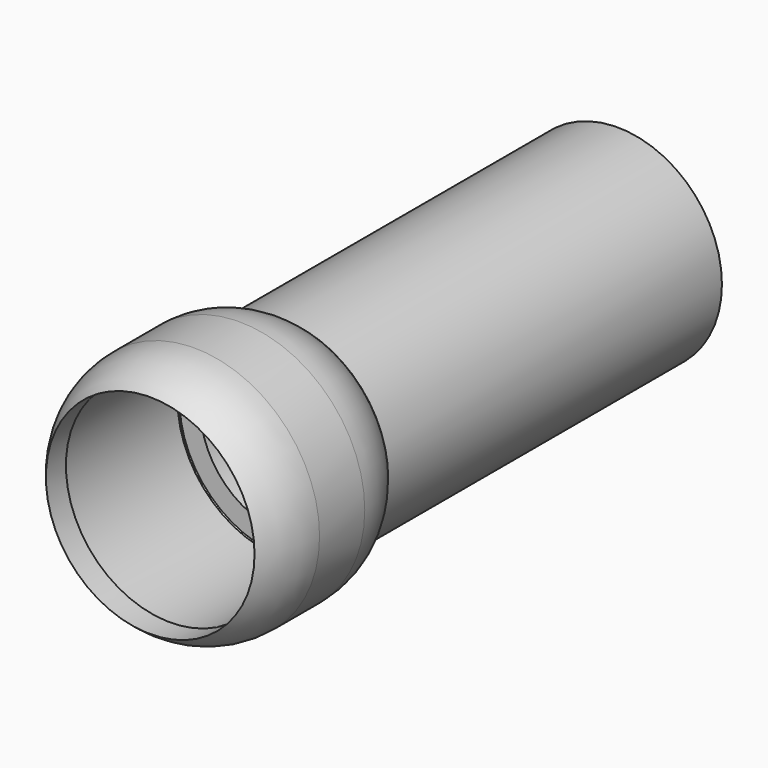
from build123d import *

# Parameters (mm, degrees)
F0_R     = 38.1
F0_R_2   = 31.75
F1_DEPTH = 50.8
F4_R     = 32.0360083413
F5_DEPTH = 43.18
F6_R     = 31.75
F6_R_2   = 25.4
F7_DEPTH = 127


# Not quite as in the source:
# - a fillet or chamfer that OpenCascade refuses, or shapes differently, is made with other operations: its cross-section is extruded or revolved along the edge and cut away or added


with BuildPart() as f1:
    # F0 (on Front) → F1 (new body)
    with BuildSketch(Plane.XZ):
        Circle(F0_R)
        Circle(F0_R_2, mode=Mode.SUBTRACT)
    extrude(amount=F1_DEPTH)

    # F2: fillet of radius 25.4 on 1 edges, made by hand

    # F2_s1 → F2_t2 (revolve, cut)
    with BuildSketch(Plane.XY):
        with BuildLine():
            ThreePointArc((38.1, -33.9994791747), (36.459524406, -42.9797352958), (31.75, -50.8))
            Line((31.75, -50.8), (38.1, -50.8))
            Line((38.1, -50.8), (38.1, -33.9994791747))
        make_face()
    revolve(axis=Axis((0, -50.8, 0), (0, -1, 0)), mode=Mode.SUBTRACT)

    # F3: fillet of radius 25.4 on 1 edges, made by hand

    # F3_s1 → F3_t2 (revolve, cut)
    with BuildSketch(Plane.XY):
        with BuildLine():
            ThreePointArc((38.1, -16.8005208253), (36.459524406, -7.8202647042), (31.75, 0))
            Line((31.75, 0), (38.1, 0))
            Line((38.1, 0), (38.1, -16.8005208253))
        make_face()
    revolve(axis=Axis((0, 0, 0), (0, -1, 0)), mode=Mode.SUBTRACT)

    # F4 (on Front) → F5 (cut)
    with BuildSketch(Plane.XZ):
        Circle(F4_R)
    extrude(amount=F5_DEPTH, mode=Mode.SUBTRACT)


with BuildPart() as f7:
    # F6 (on Front) → F7 (new body)
    with BuildSketch(Plane.XZ):
        Circle(F6_R)
        Circle(F6_R_2, mode=Mode.SUBTRACT)
    extrude(amount=-F7_DEPTH)


solid = Compound([f1.part, f7.part])
